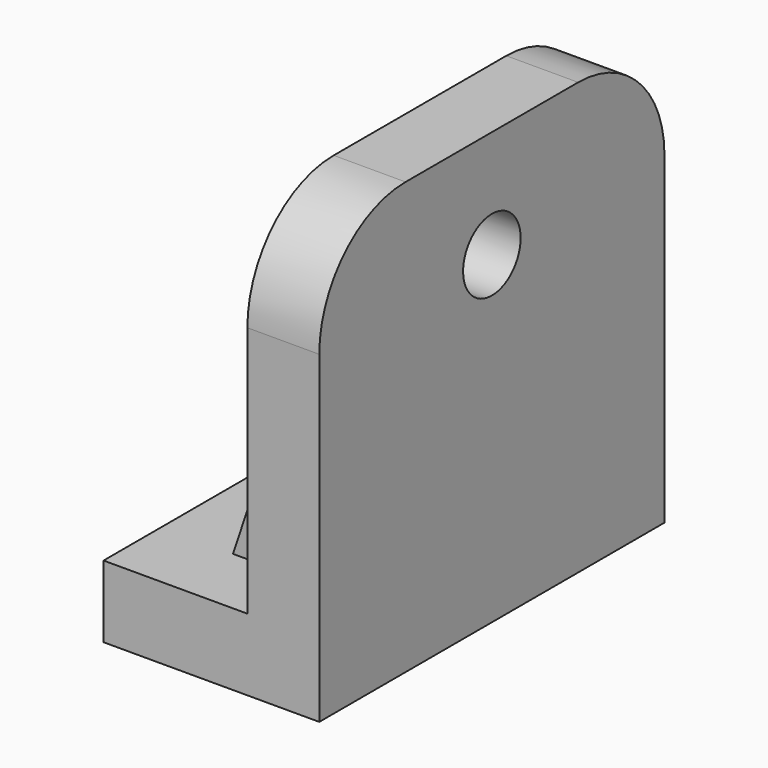
from build123d import *

# Parameters (mm, degrees)
F1_DEPTH = 76.2
F2_R     = 12.7
F3_DEPTH = 76.201
F5_DEPTH = 25.401
F6_R     = 38.1
F9_DEPTH = 6.35


# Not quite as in the source:
# - a pattern or mirror of a feature is missing from the dataset's text; its kind, count and spacing are read off the source's solid


with BuildPart() as f1:
    # F0 (on Front) → F1 (new body, symmetric)
    with BuildSketch(Plane.XZ):
        Polygon((-76.2, 0), (0, 0), (0, 152.4), (-25.4, 152.4), (-25.4, 25.4), (-76.2, 25.4), align=None)
    extrude(amount=F1_DEPTH, both=True)

    # F2 (on Right) → F3 (cut, through all)
    with BuildSketch(Plane.YZ):
        with Locations((0, 114.3)):
            Circle(F2_R)
    extrude(amount=-F3_DEPTH, mode=Mode.SUBTRACT)

    # F4 (on face) → F5 (cut, through all)
    with BuildSketch(Plane.XY.offset(25.4)):
        with BuildLine():
            Line((-76.2, 12.7), (-76.2, 0))
            Line((-76.2, 0), (-76.2, -12.7))
            Line((-76.2, -12.7), (-63.5, -12.7))
            ThreePointArc((-63.5, -12.7), (-50.8, 0), (-63.5, 12.7))
            Line((-63.5, 12.7), (-76.2, 12.7))
        make_face()
    extrude(amount=-F5_DEPTH, mode=Mode.SUBTRACT)

    # F6
    f6_edges = [f1.edges().sort_by_distance(p)[0] for p in [
        (-12.7, -76.2, 152.4),
        (-12.7, 76.2, 152.4),
    ]]
    fillet(f6_edges, radius=F6_R)

    # F8 (on offset) → F9 (join, symmetric)
    with BuildSketch(Plane.XZ.offset(44.45)):
        Polygon((-50.8, 25.4), (-25.4, 25.4), (-25.4, 101.6), align=None)
    f9 = extrude(amount=F9_DEPTH, both=True)

    # F9_copies: F9 across plane
    add(f9.mirror(Plane.ZX))


solid = f1.part
